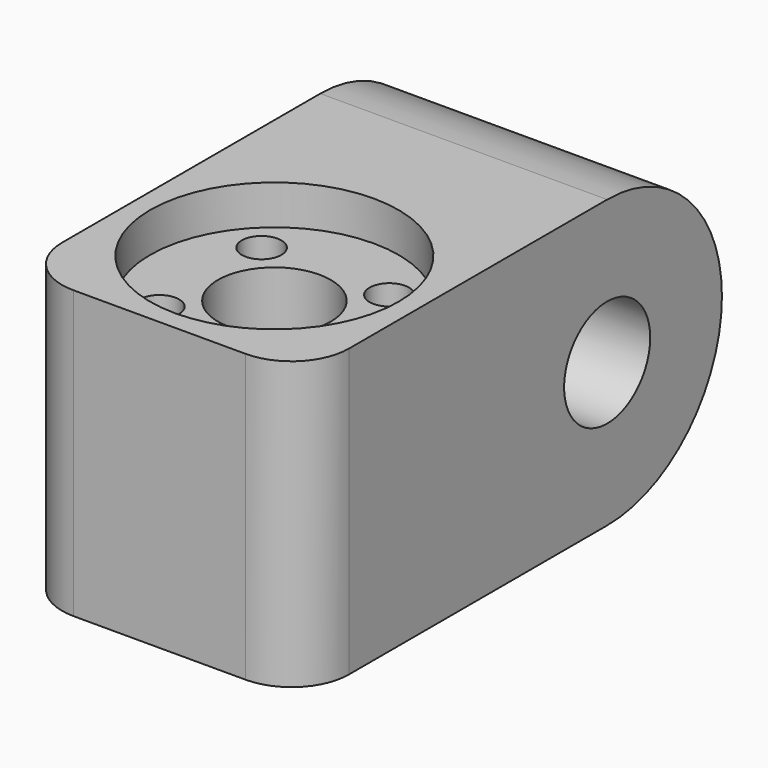
from build123d import *

# Parameters (mm, degrees)
F0_W          = 25.4
F0_H          = 25.4
F1_DEPTH      = 25.4
F2_R          = 4.7625
F3_DEPTH      = 12.7
F3_DEPTH_BACK = 12.7
F4_R          = 5.08
F5_R          = 5
F5_R_2        = 1.75
F6_DEPTH      = 25.401
F7_R          = 11
F8_DEPTH      = 3.5


with BuildPart() as f1:
    # F0 (on Top) → F1 (new body)
    with BuildSketch(Plane.XY):
        Rectangle(F0_W, F0_H)
    extrude(amount=F1_DEPTH)

    # F2 (on Right) → F3 (join, two sides)
    with BuildSketch(Plane.YZ) as f3_sk:
        with BuildLine():
            Line((12.7, 0), (20.955, 0))
            ThreePointArc((20.955, 0), (33.655, 12.7), (20.955, 25.4))
            Line((20.955, 25.4), (12.7, 25.4))
            Line((12.7, 25.4), (12.7, 0))
        make_face()
        with Locations((20.955, 12.7)):
            Circle(F2_R, mode=Mode.SUBTRACT)
    extrude(amount=F3_DEPTH)
    extrude(f3_sk.sketch, amount=-F3_DEPTH_BACK)

    # F4
    f4_edges = [f1.edges().sort_by_distance(p)[0] for p in [
        (12.7, -12.7, 12.7),
        (-12.7, -12.7, 12.7),
    ]]
    fillet(f4_edges, radius=F4_R)

    # F5 (on face) → F6 (cut, through all)
    with BuildSketch(Plane.XY.offset(25.4)):
        Circle(F5_R)
        with Locations((-5.6568542495, 5.6568542495)):
            Circle(F5_R_2)
        with Locations((5.6568542495, 5.6568542495)):
            Circle(F5_R_2)
        with BuildLine():
            ThreePointArc((3.9068542495, -5.6568542495), (5.6568542495, -7.4068542495), (7.4068542495, -5.6568542495))
            ThreePointArc((7.4068542495, -5.6568542495), (5.6568542495, -3.9068542495), (3.9068542495, -5.6568542495))
        make_face()
        with Locations((-5.6568542495, -5.6568542495)):
            Circle(F5_R_2)
    extrude(amount=-F6_DEPTH, mode=Mode.SUBTRACT)

    # F7 (on face) → F8 (cut)
    with BuildSketch(Plane.XY.offset(25.4)):
        Circle(F7_R)
    extrude(amount=-F8_DEPTH, mode=Mode.SUBTRACT)


solid = f1.part
